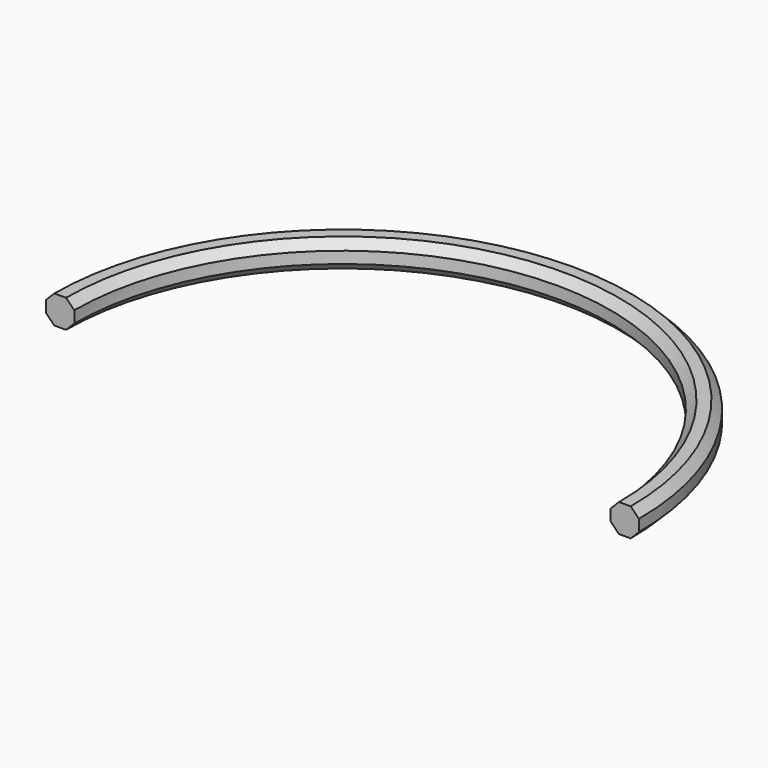
from build123d import *

# Parameters (mm, degrees)
F1_ANGLE = 180


# Not quite as in the source:
# - a feature names something its author has since deleted; it is built from what else it names


with BuildPart() as f1:
    # F0 (on Front) → F1 (revolve)
    with BuildSketch(Plane.XZ):
        Polygon((25.9260512242, 1.27), (24.8739487758, 1.27), (24.13, 0.5260512242), (24.13, -0.5260512242), (24.8739487758, -1.27), (25.9260512242, -1.27), (26.67, -0.5260512242), (26.67, 0.5260512242), align=None)
    revolve(axis=Axis((0, 0, 7.0851081982), (0, 0, 1)), revolution_arc=F1_ANGLE)


solid = f1.part
